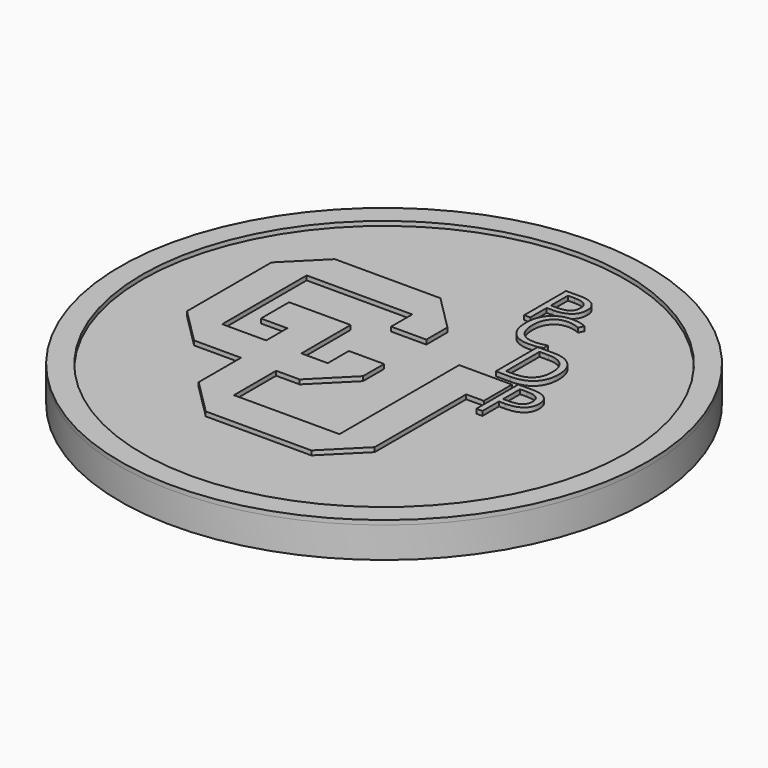
from build123d import *

# Parameters (mm, degrees)
F0_R           = 38.1
F1_DEPTH       = 3.81
F2_R           = 38.1
F2_R_2         = 34.925
F2_TEXT_SIZE   = 10.5833333333
F3_DEPTH       = 0.635
F4_R           = 38.1
F4_R_2         = 34.925
F4_TEXT_SIZE   = 10.9660010793
F4_TEXT_SIZE_2 = 8.6199095023
F5_DEPTH       = 0.635


# Not quite as in the source:
# - a feature of the source that left no trace in its solid (it failed there, or was rolled back) is left out
# - Text() gives the source's letters only with a copy of the font that has no kerning and outlines rounded to 1/6400 em; it was checked with that copy


with BuildPart() as f1:
    # F0 (on Top) → F1 (new body)
    with BuildSketch(Plane.XY):
        Circle(F0_R)
    extrude(amount=-F1_DEPTH)

    # F4 (on face) → F5 (join)
    with BuildSketch(Plane(origin=(0, 0, -3.81), x_dir=(1, 0, 0), z_dir=(0, 0, -1))):
        Circle(F4_R)
        Circle(F4_R_2, mode=Mode.SUBTRACT)
        with Locations((-8.604884998, -8.9999084315)):
            Text('2016', F4_TEXT_SIZE, font='Open Sans', font_style=FontStyle.BOLD, text_align=(TextAlign.LEFT, TextAlign.BOTTOM))
        with Locations((-13.6628926309, 2.7018362035)):
            Text('Edi Rivas', F4_TEXT_SIZE_2, font='Open Sans', font_style=FontStyle.BOLD, text_align=(TextAlign.LEFT, TextAlign.BOTTOM))
    extrude(amount=F5_DEPTH)


with BuildPart() as f3:
    # F2 (on face) → F3 (new body)
    with BuildSketch(Plane.XY):
        Circle(F2_R)
        Circle(F2_R_2, mode=Mode.SUBTRACT)
        Polygon((0, -3.81), (0, 0), (-5.08, 0), (-5.08, -3.81), (-8.89, -3.81), (-8.89, 5.08), (-13.97, 5.08), (-17.78, 5.08), (-17.78, 0), (-13.97, 0), (-13.97, -3.81), (-20.32, -3.81), (-20.32, 11.43), (-5.08, 11.43), (-5.08, 7.62), (0, 7.62), (0, 11.43), (-5.08, 16.51), (-20.32, 16.51), (-25.4, 11.43), (-25.4, 0), (-25.4, -3.81), (-20.32, -8.89), (-13.54393363, -8.89), (-13.54393363, -16.5168102831), (-8.46393363, -21.5968102831), (6.77606637, -21.5968102831), (11.85606637, -16.5168102831), (11.85606637, -0.0068102831), (14.39606637, -0.0068102831), (14.39606637, 5.0731897169), (6.77606637, 5.0731897169), (6.77606637, -16.5168102831), (-8.46393363, -16.5168102831), (-8.46393363, -8.89), (-5.08, -8.89), align=None)
        with Locations((3.8479368848, 19.1728020701)):
            Text('P', F2_TEXT_SIZE, font='Open Sans', text_align=(TextAlign.LEFT, TextAlign.BOTTOM))
        with Locations((5.5351379276, 14.0928020701)):
            Text('C', F2_TEXT_SIZE, font='Open Sans', text_align=(TextAlign.LEFT, TextAlign.BOTTOM))
        with Locations((9.9073775109, 6.4728020701)):
            Text('D', F2_TEXT_SIZE, font='Open Sans', text_align=(TextAlign.LEFT, TextAlign.BOTTOM))
        with Locations((13.90505312, -2.0257459943)):
            Text('P', F2_TEXT_SIZE, font='Open Sans', text_align=(TextAlign.LEFT, TextAlign.BOTTOM))
    extrude(amount=F3_DEPTH)


solid = Compound([f1.part, f3.part])
